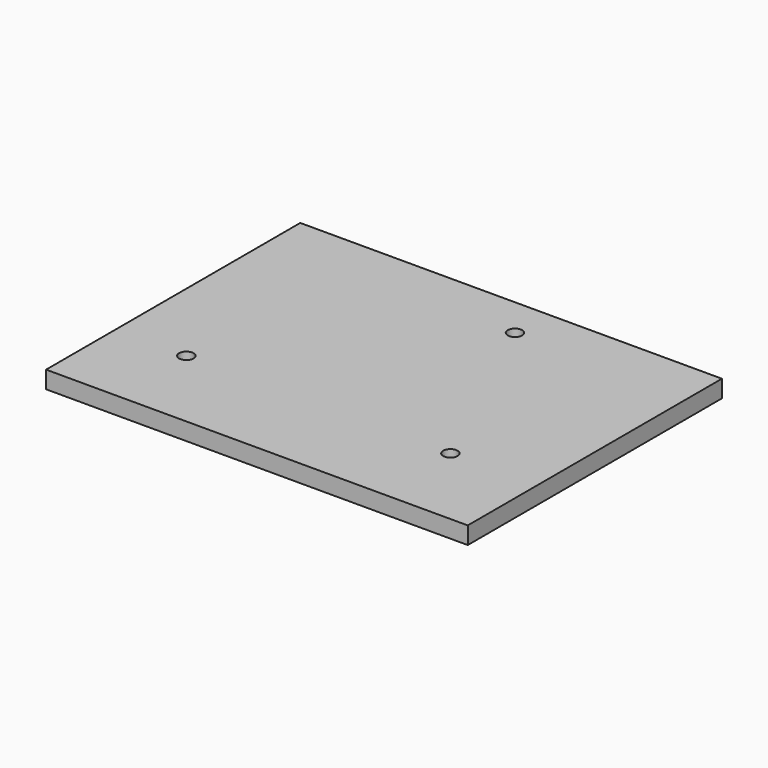
from build123d import *

# Parameters (mm, degrees)
F0_W     = 73
F0_H     = 55
F0_R     = 3.5
F0_R_2   = 1.25
F1_DEPTH = 3


# Not quite as in the source:
# - a feature names something its author has since deleted; it is built from what else it names


with BuildPart() as f1:
    # F0 (on Top) → F1 (new body)
    with BuildSketch(Plane.XY):
        with Locations((17.8632747996, -5.3606596088)):
            Rectangle(F0_W, F0_H)
        with Locations((-6.3567252004, -17.8606596088)):
            Circle(F0_R, mode=Mode.SUBTRACT)
        with BuildLine():
            ThreePointArc((39.3632747996, -14.3606596088), (41.8381485337, -15.3857858747), (42.8632747996, -17.8606596088))
            ThreePointArc((42.8632747996, -17.8606596088), (41.8381485337, -20.335533343), (39.3632747996, -21.3606596088))
            ThreePointArc((39.3632747996, -21.3606596088), (35.8632747996, -17.8606596088), (39.3632747996, -14.3606596088))
        make_face(mode=Mode.SUBTRACT)
        with Locations((24.1232747996, 15.1593403912)):
            Circle(F0_R, mode=Mode.SUBTRACT)
        with Locations((24.1232747996, 15.1593403912)):
            Circle(F0_R)
        with Locations((24.1232747996, 15.1593403912)):
            Circle(F0_R_2, mode=Mode.SUBTRACT)
        with BuildLine():
            ThreePointArc((39.3632747996, -21.3606596088), (41.8381485337, -20.335533343), (42.8632747996, -17.8606596088))
            ThreePointArc((42.8632747996, -17.8606596088), (41.8381485337, -15.3857858747), (39.3632747996, -14.3606596088))
            ThreePointArc((39.3632747996, -14.3606596088), (35.8632747996, -17.8606596088), (39.3632747996, -21.3606596088))
        make_face()
        with Locations((39.3632747996, -17.8606596088)):
            Circle(F0_R_2, mode=Mode.SUBTRACT)
        with Locations((-6.3567252004, -17.8606596088)):
            Circle(F0_R)
        with Locations((-6.3567252004, -17.8606596088)):
            Circle(F0_R_2, mode=Mode.SUBTRACT)
    extrude(amount=-F1_DEPTH)


solid = f1.part
